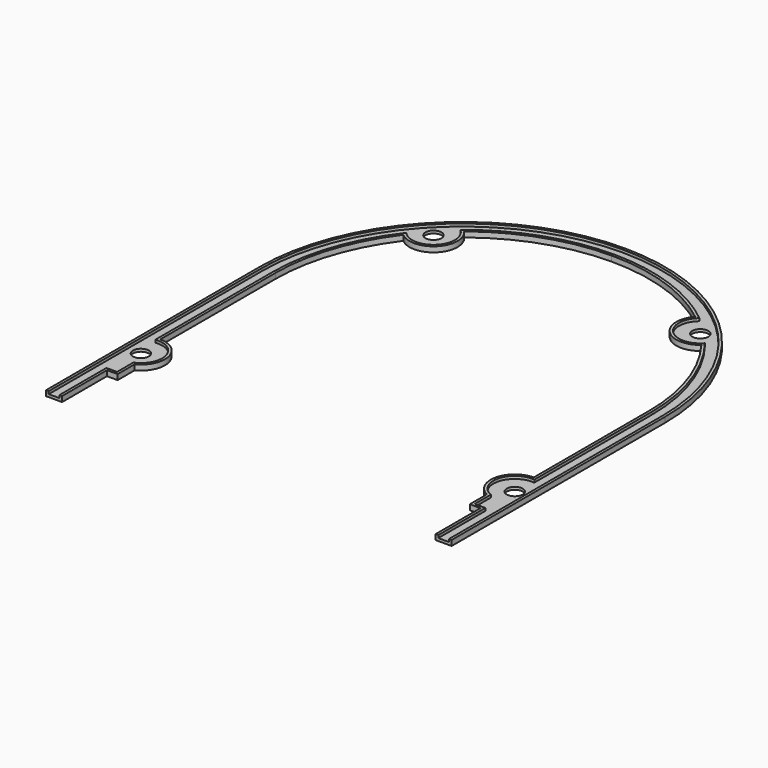
from build123d import *

# Parameters (mm, degrees)
F0_R     = 3
F1_DEPTH = 2
F2_T     = -1
F4_W     = 4
F4_H     = 1
F4_R     = 4
F4_R_2   = 3
F5_DEPTH = 1


# Not quite as in the source:
# - a feature of the source that left no trace in its solid (it failed there, or was rolled back) is left out


with BuildPart() as f1:
    # F0 (on Top) → F1 (new body)
    with BuildSketch(Plane.XY):
        with BuildLine():
            ThreePointArc((76, 31), (0, 107), (-76, 31))
            Line((-76, 31), (-76, -31))
            Line((-76, -31), (-76, -69))
            Line((-76, -69), (-70, -69))
            Line((-70, -69), (-70, -47.9877756238))
            Line((-70, -47.9877756238), (-66, -47.9877756238))
            Line((-66, -47.9877756238), (-66, -40.0317243588))
            ThreePointArc((-66, -40.0317243588), (-61.2993566139, -29.9422610746), (-70, -23.00020646))
            Line((-70, -23.00020646), (-70, 31))
            ThreePointArc((-70, 31), (-66.3741952073, 53.2365962005), (-55.8723939833, 73.1696050559))
            ThreePointArc((-55.8723939833, 73.1696050559), (-43.5714285714, 73.6911069456), (-43.3010754044, 86.0001533527))
            ThreePointArc((-43.3010754044, 86.0001533527), (-22.9127613494, 97.1438233499), (0, 101))
            ThreePointArc((0, 101), (22.9127613494, 97.1438233499), (43.3010754044, 86.0001533527))
            ThreePointArc((43.3010754044, 86.0001533527), (43.5714285714, 73.6911069456), (55.8723939833, 73.1696050559))
            ThreePointArc((55.8723939833, 73.1696050559), (66.3741952073, 53.2365962005), (70, 31))
            Line((70, 31), (70, -23.00020646))
            ThreePointArc((70, -23.00020646), (61.2993566139, -29.9422610746), (66, -40.0317243588))
            Line((66, -40.0317243588), (66, -47.9877756238))
            Line((66, -47.9877756238), (70, -47.9877756238))
            Line((70, -47.9877756238), (70, -69))
            Line((70, -69), (76, -69))
            Line((76, -69), (76, -31))
            Line((76, -31), (76, 31))
        make_face()
        with Locations((-70.0609609485, -32)):
            Circle(F0_R, mode=Mode.SUBTRACT)
        with Locations((70.0609609485, -32)):
            Circle(F0_R, mode=Mode.SUBTRACT)
        with Locations((-50, 79.9897948557)):
            Circle(F0_R, mode=Mode.SUBTRACT)
        with Locations((50, 79.9897948557)):
            Circle(F0_R, mode=Mode.SUBTRACT)
    extrude(amount=F1_DEPTH)

    # F2
    f2_openings = [f1.faces().sort_by_distance(p)[0] for p in [
        (0, 104.674489, 2),
    ]]
    offset(amount=F2_T, openings=f2_openings, kind=Kind.INTERSECTION)

    # F4 (on face) → F5 (cut)
    with BuildSketch(Plane.XY.offset(2)):
        with Locations((73, -68.5)):
            Rectangle(F4_W, F4_H)
        with Locations((-73, -68.5)):
            Rectangle(F4_W, F4_H)
        with Locations((-70.0609609485, -32)):
            Circle(F4_R)
        with Locations((-70.0609609485, -32)):
            Circle(F4_R_2, mode=Mode.SUBTRACT)
        with Locations((70.0609609485, -32)):
            Circle(F4_R)
        with Locations((70.0609609485, -32)):
            Circle(F4_R_2, mode=Mode.SUBTRACT)
        with Locations((-50, 79.9897948557)):
            Circle(F4_R)
        with Locations((-50, 79.9897948557)):
            Circle(F4_R_2, mode=Mode.SUBTRACT)
        with Locations((50, 79.9897948557)):
            Circle(F4_R)
        with Locations((50, 79.9897948557)):
            Circle(F4_R_2, mode=Mode.SUBTRACT)
    extrude(amount=-F5_DEPTH, mode=Mode.SUBTRACT)


solid = f1.part
